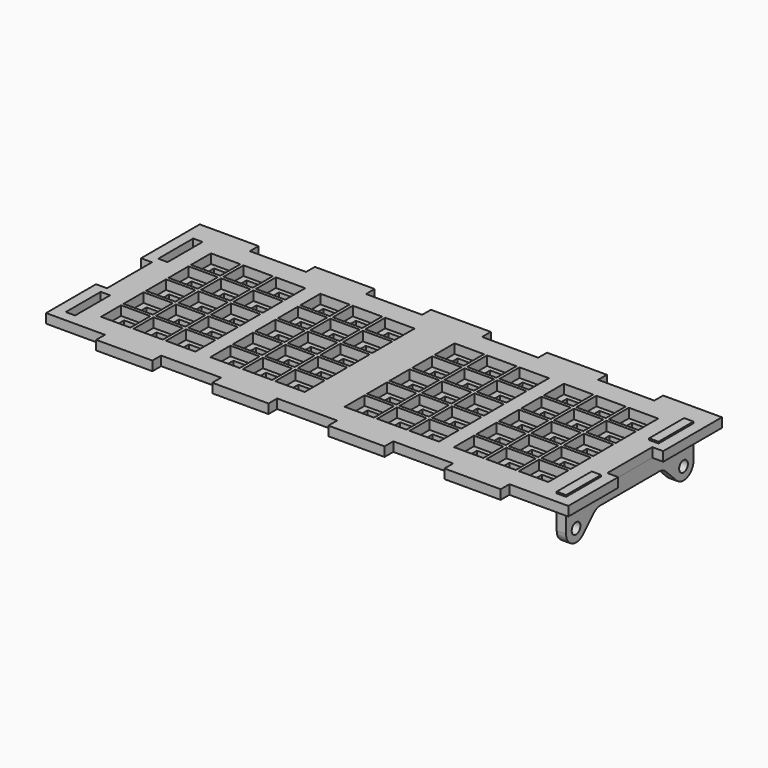
from build123d import *

# Parameters (mm, degrees)
F0_W     = 147.2
F0_H     = 49
F0_W_2   = 5.2
F0_H_2   = 5.2
F1_DEPTH = 3
F2_W     = 167.2
F2_H     = 65
F2_W_2   = 9.4
F2_H_2   = 8
F3_DEPTH = 3
F4_W     = 3
F4_H     = 14
F4_W_2   = 3.5
F4_H_2   = 18
F4_W_3   = 18
F4_H_3   = 3.5
F4_W_4   = 18.8466580786
F4_W_5   = 19.1688946143
F5_DEPTH = 25
F6_R     = 1.75
F7_DEPTH = 3
F8_R     = 3.99999


# Not quite as in the source:
# - a fillet or chamfer is up to 0.001 mm smaller than in the source, because OpenCascade refuses the exact size


with BuildPart() as f1:
    # F0 (on Top) → F1 (new body)
    with BuildSketch(Plane.XY):
        with Locations((73.6, 24.5)):
            Rectangle(F0_W, F0_H)
        with Locations((6.7, 6.5)):
            Rectangle(F0_W_2, F0_H_2, mode=Mode.SUBTRACT)
        with Locations((17.1, 6.5)):
            Rectangle(F0_W_2, F0_H_2, mode=Mode.SUBTRACT)
        with Locations((27.5, 6.5)):
            Rectangle(F0_W_2, F0_H_2, mode=Mode.SUBTRACT)
        with Locations((41.7, 6.5)):
            Rectangle(F0_W_2, F0_H_2, mode=Mode.SUBTRACT)
        with Locations((52.1, 6.5)):
            Rectangle(F0_W_2, F0_H_2, mode=Mode.SUBTRACT)
        with Locations((62.5, 6.5)):
            Rectangle(F0_W_2, F0_H_2, mode=Mode.SUBTRACT)
        with Locations((6.7, 15.5)):
            Rectangle(F0_W_2, F0_H_2, mode=Mode.SUBTRACT)
        with Locations((17.1, 15.5)):
            Rectangle(F0_W_2, F0_H_2, mode=Mode.SUBTRACT)
        with Locations((27.5, 15.5)):
            Rectangle(F0_W_2, F0_H_2, mode=Mode.SUBTRACT)
        with Locations((6.7, 24.5)):
            Rectangle(F0_W_2, F0_H_2, mode=Mode.SUBTRACT)
        with Locations((17.1, 24.5)):
            Rectangle(F0_W_2, F0_H_2, mode=Mode.SUBTRACT)
        with Locations((27.5, 24.5)):
            Rectangle(F0_W_2, F0_H_2, mode=Mode.SUBTRACT)
        with Locations((41.7, 15.5)):
            Rectangle(F0_W_2, F0_H_2, mode=Mode.SUBTRACT)
        with Locations((52.1, 15.5)):
            Rectangle(F0_W_2, F0_H_2, mode=Mode.SUBTRACT)
        with Locations((62.5, 15.5)):
            Rectangle(F0_W_2, F0_H_2, mode=Mode.SUBTRACT)
        with Locations((41.7, 24.5)):
            Rectangle(F0_W_2, F0_H_2, mode=Mode.SUBTRACT)
        with Locations((52.1, 24.5)):
            Rectangle(F0_W_2, F0_H_2, mode=Mode.SUBTRACT)
        with Locations((62.5, 24.5)):
            Rectangle(F0_W_2, F0_H_2, mode=Mode.SUBTRACT)
        with Locations((84.7, 6.5)):
            Rectangle(F0_W_2, F0_H_2, mode=Mode.SUBTRACT)
        with Locations((95.1, 6.5)):
            Rectangle(F0_W_2, F0_H_2, mode=Mode.SUBTRACT)
        with Locations((105.5, 6.5)):
            Rectangle(F0_W_2, F0_H_2, mode=Mode.SUBTRACT)
        with Locations((119.7, 6.5)):
            Rectangle(F0_W_2, F0_H_2, mode=Mode.SUBTRACT)
        with Locations((130.1, 6.5)):
            Rectangle(F0_W_2, F0_H_2, mode=Mode.SUBTRACT)
        with Locations((140.5, 6.5)):
            Rectangle(F0_W_2, F0_H_2, mode=Mode.SUBTRACT)
        with Locations((84.7, 15.5)):
            Rectangle(F0_W_2, F0_H_2, mode=Mode.SUBTRACT)
        with Locations((95.1, 15.5)):
            Rectangle(F0_W_2, F0_H_2, mode=Mode.SUBTRACT)
        with Locations((105.5, 15.5)):
            Rectangle(F0_W_2, F0_H_2, mode=Mode.SUBTRACT)
        with Locations((84.7, 24.5)):
            Rectangle(F0_W_2, F0_H_2, mode=Mode.SUBTRACT)
        with Locations((95.1, 24.5)):
            Rectangle(F0_W_2, F0_H_2, mode=Mode.SUBTRACT)
        with Locations((105.5, 24.5)):
            Rectangle(F0_W_2, F0_H_2, mode=Mode.SUBTRACT)
        with Locations((119.7, 15.5)):
            Rectangle(F0_W_2, F0_H_2, mode=Mode.SUBTRACT)
        with Locations((130.1, 15.5)):
            Rectangle(F0_W_2, F0_H_2, mode=Mode.SUBTRACT)
        with Locations((140.5, 15.5)):
            Rectangle(F0_W_2, F0_H_2, mode=Mode.SUBTRACT)
        with Locations((119.7, 24.5)):
            Rectangle(F0_W_2, F0_H_2, mode=Mode.SUBTRACT)
        with Locations((130.1, 24.5)):
            Rectangle(F0_W_2, F0_H_2, mode=Mode.SUBTRACT)
        with Locations((140.5, 24.5)):
            Rectangle(F0_W_2, F0_H_2, mode=Mode.SUBTRACT)
        with Locations((6.7, 33.5)):
            Rectangle(F0_W_2, F0_H_2, mode=Mode.SUBTRACT)
        with Locations((17.1, 33.5)):
            Rectangle(F0_W_2, F0_H_2, mode=Mode.SUBTRACT)
        with Locations((27.5, 33.5)):
            Rectangle(F0_W_2, F0_H_2, mode=Mode.SUBTRACT)
        with Locations((41.7, 33.5)):
            Rectangle(F0_W_2, F0_H_2, mode=Mode.SUBTRACT)
        with Locations((52.1, 33.5)):
            Rectangle(F0_W_2, F0_H_2, mode=Mode.SUBTRACT)
        with Locations((62.5, 33.5)):
            Rectangle(F0_W_2, F0_H_2, mode=Mode.SUBTRACT)
        with Locations((6.7, 42.5)):
            Rectangle(F0_W_2, F0_H_2, mode=Mode.SUBTRACT)
        with Locations((17.1, 42.5)):
            Rectangle(F0_W_2, F0_H_2, mode=Mode.SUBTRACT)
        with Locations((27.5, 42.5)):
            Rectangle(F0_W_2, F0_H_2, mode=Mode.SUBTRACT)
        with Locations((41.7, 42.5)):
            Rectangle(F0_W_2, F0_H_2, mode=Mode.SUBTRACT)
        with Locations((52.1, 42.5)):
            Rectangle(F0_W_2, F0_H_2, mode=Mode.SUBTRACT)
        with Locations((62.5, 42.5)):
            Rectangle(F0_W_2, F0_H_2, mode=Mode.SUBTRACT)
        with Locations((84.7, 33.5)):
            Rectangle(F0_W_2, F0_H_2, mode=Mode.SUBTRACT)
        with Locations((95.1, 33.5)):
            Rectangle(F0_W_2, F0_H_2, mode=Mode.SUBTRACT)
        with Locations((105.5, 33.5)):
            Rectangle(F0_W_2, F0_H_2, mode=Mode.SUBTRACT)
        with Locations((119.7, 33.5)):
            Rectangle(F0_W_2, F0_H_2, mode=Mode.SUBTRACT)
        with Locations((130.1, 33.5)):
            Rectangle(F0_W_2, F0_H_2, mode=Mode.SUBTRACT)
        with Locations((140.5, 33.5)):
            Rectangle(F0_W_2, F0_H_2, mode=Mode.SUBTRACT)
        with Locations((84.7, 42.5)):
            Rectangle(F0_W_2, F0_H_2, mode=Mode.SUBTRACT)
        with Locations((95.1, 42.5)):
            Rectangle(F0_W_2, F0_H_2, mode=Mode.SUBTRACT)
        with Locations((105.5, 42.5)):
            Rectangle(F0_W_2, F0_H_2, mode=Mode.SUBTRACT)
        with Locations((119.7, 42.5)):
            Rectangle(F0_W_2, F0_H_2, mode=Mode.SUBTRACT)
        with Locations((130.1, 42.5)):
            Rectangle(F0_W_2, F0_H_2, mode=Mode.SUBTRACT)
        with Locations((140.5, 42.5)):
            Rectangle(F0_W_2, F0_H_2, mode=Mode.SUBTRACT)
    extrude(amount=F1_DEPTH)


with BuildPart() as f3:
    # F2 (on face) → F3 (new body)
    with BuildSketch(Plane.XY.offset(3)):
        with Locations((73.6, 24.5)):
            Rectangle(F2_W, F2_H)
        with Locations((6.7, 6.5)):
            Rectangle(F2_W_2, F2_H_2, mode=Mode.SUBTRACT)
        with Locations((17.1, 6.5)):
            Rectangle(F2_W_2, F2_H_2, mode=Mode.SUBTRACT)
        with Locations((27.5, 6.5)):
            Rectangle(F2_W_2, F2_H_2, mode=Mode.SUBTRACT)
        with Locations((41.7, 6.5)):
            Rectangle(F2_W_2, F2_H_2, mode=Mode.SUBTRACT)
        with Locations((52.1, 6.5)):
            Rectangle(F2_W_2, F2_H_2, mode=Mode.SUBTRACT)
        with Locations((62.5, 6.5)):
            Rectangle(F2_W_2, F2_H_2, mode=Mode.SUBTRACT)
        with Locations((6.7, 15.5)):
            Rectangle(F2_W_2, F2_H_2, mode=Mode.SUBTRACT)
        with Locations((17.1, 15.5)):
            Rectangle(F2_W_2, F2_H_2, mode=Mode.SUBTRACT)
        with Locations((27.5, 15.5)):
            Rectangle(F2_W_2, F2_H_2, mode=Mode.SUBTRACT)
        with Locations((41.7, 15.5)):
            Rectangle(F2_W_2, F2_H_2, mode=Mode.SUBTRACT)
        with Locations((52.1, 15.5)):
            Rectangle(F2_W_2, F2_H_2, mode=Mode.SUBTRACT)
        with Locations((62.5, 15.5)):
            Rectangle(F2_W_2, F2_H_2, mode=Mode.SUBTRACT)
        with Locations((84.7, 6.5)):
            Rectangle(F2_W_2, F2_H_2, mode=Mode.SUBTRACT)
        with Locations((95.1, 6.5)):
            Rectangle(F2_W_2, F2_H_2, mode=Mode.SUBTRACT)
        with Locations((105.5, 6.5)):
            Rectangle(F2_W_2, F2_H_2, mode=Mode.SUBTRACT)
        with Locations((119.7, 6.5)):
            Rectangle(F2_W_2, F2_H_2, mode=Mode.SUBTRACT)
        with Locations((130.1, 6.5)):
            Rectangle(F2_W_2, F2_H_2, mode=Mode.SUBTRACT)
        with Locations((140.5, 6.5)):
            Rectangle(F2_W_2, F2_H_2, mode=Mode.SUBTRACT)
        with Locations((84.7, 15.5)):
            Rectangle(F2_W_2, F2_H_2, mode=Mode.SUBTRACT)
        with Locations((95.1, 15.5)):
            Rectangle(F2_W_2, F2_H_2, mode=Mode.SUBTRACT)
        with Locations((105.5, 15.5)):
            Rectangle(F2_W_2, F2_H_2, mode=Mode.SUBTRACT)
        with Locations((119.7, 15.5)):
            Rectangle(F2_W_2, F2_H_2, mode=Mode.SUBTRACT)
        with Locations((130.1, 15.5)):
            Rectangle(F2_W_2, F2_H_2, mode=Mode.SUBTRACT)
        with Locations((140.5, 15.5)):
            Rectangle(F2_W_2, F2_H_2, mode=Mode.SUBTRACT)
        with Locations((6.7, 24.5)):
            Rectangle(F2_W_2, F2_H_2, mode=Mode.SUBTRACT)
        with Locations((17.1, 24.5)):
            Rectangle(F2_W_2, F2_H_2, mode=Mode.SUBTRACT)
        with Locations((27.5, 24.5)):
            Rectangle(F2_W_2, F2_H_2, mode=Mode.SUBTRACT)
        with Locations((6.7, 33.5)):
            Rectangle(F2_W_2, F2_H_2, mode=Mode.SUBTRACT)
        with Locations((17.1, 33.5)):
            Rectangle(F2_W_2, F2_H_2, mode=Mode.SUBTRACT)
        with Locations((27.5, 33.5)):
            Rectangle(F2_W_2, F2_H_2, mode=Mode.SUBTRACT)
        with Locations((41.7, 24.5)):
            Rectangle(F2_W_2, F2_H_2, mode=Mode.SUBTRACT)
        with Locations((52.1, 24.5)):
            Rectangle(F2_W_2, F2_H_2, mode=Mode.SUBTRACT)
        with Locations((62.5, 24.5)):
            Rectangle(F2_W_2, F2_H_2, mode=Mode.SUBTRACT)
        with Locations((41.7, 33.5)):
            Rectangle(F2_W_2, F2_H_2, mode=Mode.SUBTRACT)
        with Locations((52.1, 33.5)):
            Rectangle(F2_W_2, F2_H_2, mode=Mode.SUBTRACT)
        with Locations((62.5, 33.5)):
            Rectangle(F2_W_2, F2_H_2, mode=Mode.SUBTRACT)
        with Locations((6.7, 42.5)):
            Rectangle(F2_W_2, F2_H_2, mode=Mode.SUBTRACT)
        with Locations((17.1, 42.5)):
            Rectangle(F2_W_2, F2_H_2, mode=Mode.SUBTRACT)
        with Locations((27.5, 42.5)):
            Rectangle(F2_W_2, F2_H_2, mode=Mode.SUBTRACT)
        with Locations((41.7, 42.5)):
            Rectangle(F2_W_2, F2_H_2, mode=Mode.SUBTRACT)
        with Locations((52.1, 42.5)):
            Rectangle(F2_W_2, F2_H_2, mode=Mode.SUBTRACT)
        with Locations((62.5, 42.5)):
            Rectangle(F2_W_2, F2_H_2, mode=Mode.SUBTRACT)
        with Locations((84.7, 24.5)):
            Rectangle(F2_W_2, F2_H_2, mode=Mode.SUBTRACT)
        with Locations((95.1, 24.5)):
            Rectangle(F2_W_2, F2_H_2, mode=Mode.SUBTRACT)
        with Locations((105.5, 24.5)):
            Rectangle(F2_W_2, F2_H_2, mode=Mode.SUBTRACT)
        with Locations((84.7, 33.5)):
            Rectangle(F2_W_2, F2_H_2, mode=Mode.SUBTRACT)
        with Locations((95.1, 33.5)):
            Rectangle(F2_W_2, F2_H_2, mode=Mode.SUBTRACT)
        with Locations((105.5, 33.5)):
            Rectangle(F2_W_2, F2_H_2, mode=Mode.SUBTRACT)
        with Locations((119.7, 24.5)):
            Rectangle(F2_W_2, F2_H_2, mode=Mode.SUBTRACT)
        with Locations((130.1, 24.5)):
            Rectangle(F2_W_2, F2_H_2, mode=Mode.SUBTRACT)
        with Locations((140.5, 24.5)):
            Rectangle(F2_W_2, F2_H_2, mode=Mode.SUBTRACT)
        with Locations((119.7, 33.5)):
            Rectangle(F2_W_2, F2_H_2, mode=Mode.SUBTRACT)
        with Locations((130.1, 33.5)):
            Rectangle(F2_W_2, F2_H_2, mode=Mode.SUBTRACT)
        with Locations((140.5, 33.5)):
            Rectangle(F2_W_2, F2_H_2, mode=Mode.SUBTRACT)
        with Locations((84.7, 42.5)):
            Rectangle(F2_W_2, F2_H_2, mode=Mode.SUBTRACT)
        with Locations((95.1, 42.5)):
            Rectangle(F2_W_2, F2_H_2, mode=Mode.SUBTRACT)
        with Locations((105.5, 42.5)):
            Rectangle(F2_W_2, F2_H_2, mode=Mode.SUBTRACT)
        with Locations((119.7, 42.5)):
            Rectangle(F2_W_2, F2_H_2, mode=Mode.SUBTRACT)
        with Locations((130.1, 42.5)):
            Rectangle(F2_W_2, F2_H_2, mode=Mode.SUBTRACT)
        with Locations((140.5, 42.5)):
            Rectangle(F2_W_2, F2_H_2, mode=Mode.SUBTRACT)
    extrude(amount=F3_DEPTH)

    # F4 (on face) → F5 (cut)
    with BuildSketch(Plane.XY.offset(6)):
        with Locations((-5, 43)):
            Rectangle(F4_W, F4_H)
        with Locations((-5, 6)):
            Rectangle(F4_W, F4_H)
        with Locations((152.2, 43)):
            Rectangle(F4_W, F4_H)
        with Locations((-8.25, 24.5)):
            Rectangle(F4_W_2, F4_H_2)
        with Locations((155.45, 24.5)):
            Rectangle(F4_W_2, F4_H_2)
        with Locations((17.8466580786, 55.25)):
            Rectangle(F4_W_3, F4_H_3)
        with Locations((55.0155526929, 55.25)):
            Rectangle(F4_W_3, F4_H_3)
        with Locations((92.1844473071, 55.25)):
            Rectangle(F4_W_3, F4_H_3)
        with Locations((129.3533419214, 55.25)):
            Rectangle(F4_W_3, F4_H_3)
        with Locations((-0.5766709607, -6.25)):
            Rectangle(F4_W_4, F4_H_3)
        with Locations((36.4311053857, -6.25)):
            Rectangle(F4_W_5, F4_H_3)
        with Locations((73.6, -6.25)):
            Rectangle(F4_W_5, F4_H_3)
        with Locations((110.7688946143, -6.25)):
            Rectangle(F4_W_5, F4_H_3)
        with Locations((147.7766709607, -6.25)):
            Rectangle(F4_W_4, F4_H_3)
        with Locations((152.2, 6)):
            Rectangle(F4_W, F4_H)
    extrude(amount=-F5_DEPTH, mode=Mode.SUBTRACT)


with BuildPart() as f7:
    # F6 (on face) → F7 (new body)
    with BuildSketch(Plane.YZ.offset(150.7)):
        Polygon((-1, 6.5), (-1, -8.5), (4.6568542495, -8.5), (11.1568542495, -2), (37.8431457505, -2), (44.3431457505, -8.5), (50, -8.5), (50, 6.5), (36, 6.5), (36, 3), (13, 3), (13, 6.5), align=None)
        with Locations((3, -4.5)):
            Circle(F6_R, mode=Mode.SUBTRACT)
        with Locations((46, -4.5)):
            Circle(F6_R, mode=Mode.SUBTRACT)
    extrude(amount=F7_DEPTH)

    # F8 (radius 4 in the source; OpenCascade refuses exactly that, so slightly less here)
    f8_edges = [f7.edges().sort_by_distance(p)[0] for p in [
        (152.2, -1, -8.5),
        (152.2, 4.656854, -8.5),
        (152.2, 11.156854, -2),
        (152.2, 37.843146, -2),
        (152.2, 44.343146, -8.5),
        (152.2, 50, -8.5),
    ]]
    fillet(f8_edges, radius=F8_R)


solid = Compound([f1.part, f3.part, f7.part])
